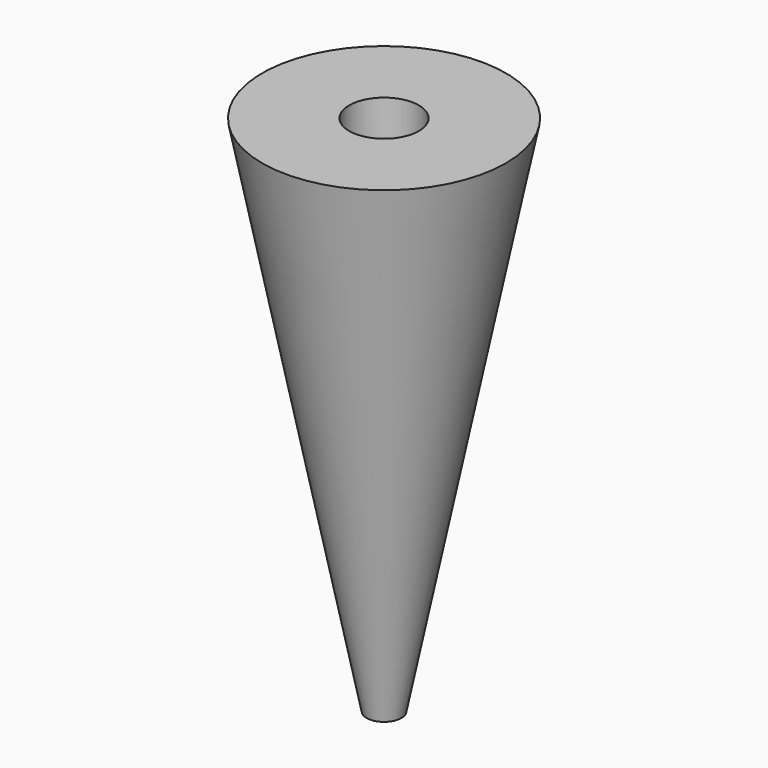
from build123d import *

# Parameters (mm, degrees)
F0_R     = 7
F1_DEPTH = 30
F3_D     = 4
F3_DEPTH = 10
F3_TIP   = 1.2017212381
F4_SIZE2 = 5.99999
F4_SIZE  = 29.99999


# Not quite as in the source:
# - a fillet or chamfer is up to 0.001 mm smaller than in the source, because OpenCascade refuses the exact size


with BuildPart() as f1:
    # F0 (on Top) → F1 (new body)
    with BuildSketch(Plane.XY):
        Circle(F0_R)
    extrude(amount=F1_DEPTH)

    # F3
    with Locations(Plane.XY.offset(30)):
        with Locations((0, 0)):
            Hole(F3_D / 2, depth=F3_DEPTH)
            with Locations((0, 0, -(F3_DEPTH + F3_TIP / 2))):  # 118° drill point
                Cone(0, F3_D / 2, F3_TIP, mode=Mode.SUBTRACT)

    # F4 (size 30 and 6 in the source; OpenCascade refuses exactly that, so slightly less here)
    f4_edges = [f1.edges().sort_by_distance(p)[0] for p in [
        (-7, 0, 0),
    ]]
    f4_side = f1.faces().sort_by_distance((-7, 0, 15))[0]
    chamfer(f4_edges, length=F4_SIZE, length2=F4_SIZE2, reference=f4_side)


solid = f1.part
